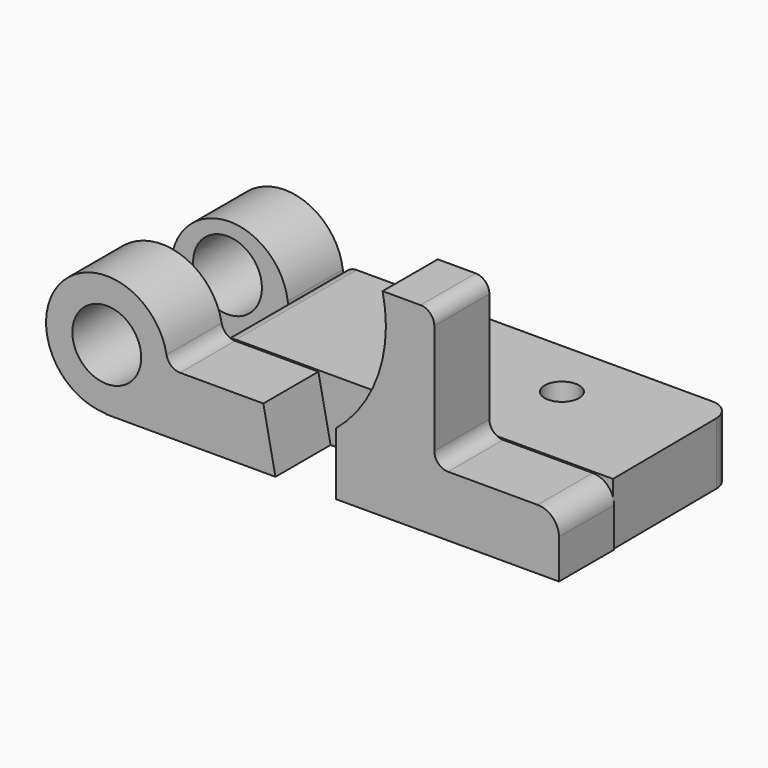
from build123d import *

# Parameters (mm, degrees)
F1_DEPTH      = 25.4
F2_R          = 22.395901736
F3_DEPTH      = 25.4
F5_DEPTH      = 22.86
F6_R          = 6.35
F7_DEPTH      = 22.861
F9_DEPTH      = 25.4
F10_T1_DEPTH  = 25.4
F10_T3_DEPTH  = 50.8
F11_R         = 21.59
F12_DEPTH     = 25.4
F13_T4_DEPTH  = 68.3456632912
F13_S5_R      = 21.59
F13_T6_DEPTH  = 36
F13_T11_DEPTH = 68.3456632912
F13_S12_R     = 21.59
F13_T13_DEPTH = 36
F13_T18_DEPTH = 68.3456632912
F13_S19_R     = 21.59
F13_T20_DEPTH = 36
F14_R         = 12.7
F15_DEPTH     = 81.0466632912


# Not quite as in the source:
# - a fillet or chamfer that OpenCascade refuses, or shapes differently, is made with other operations: its cross-section is extruded or revolved along the edge and cut away or added


with BuildPart() as f1:
    # F0 (on Front) → F1 (new body)
    with BuildSketch(Plane.XZ):
        with BuildLine():
            Line((-62.5702434896, 0), (104.5470208636, 0))
            Line((104.5470208636, 0), (104.5470208636, 14.478))
            ThreePointArc((104.5470208636, 14.478), (102.2407796587, 20.0457587951), (96.6730208636, 22.352))
            Line((96.6730208636, 22.352), (58.5730208636, 22.352))
            Line((58.5730208636, 22.352), (58.5730208636, 73.152))
            Line((58.5730208636, 73.152), (39.5230208636, 73.152))
            ThreePointArc((39.5230208636, 73.152), (37.7930667188, 45.1601637849), (21.4736518763, 22.352))
            Line((21.4736518763, 22.352), (-62.5702434896, 22.352))
            Line((-62.5702434896, 22.352), (-62.5702434896, 0))
        make_face()
    extrude(amount=F1_DEPTH)

    # F2 (on Front) → F3 (join)
    with BuildSketch(Plane.XZ):
        with Locations((-62.223136425, 22.609276697)):
            Circle(F2_R)
    extrude(amount=F3_DEPTH)

    # F4 (on Top) → F5 (join)
    with BuildSketch(Plane.XY):
        with BuildLine():
            Line((-40.0024205446, 55.6456632912), (-40.0024205446, 0))
            Line((-40.0024205446, 0), (104.1451707114, 0))
            Line((104.1451707114, 0), (103.7883380443, 48.0822120633))
            ThreePointArc((103.7883380443, 48.0822120633), (101.536671306, 53.4337730184), (96.1685478742, 55.6456632912))
            Line((96.1685478742, 55.6456632912), (-40.0024205446, 55.6456632912))
        make_face()
    extrude(amount=F5_DEPTH)

    # F6 (on face) → F7 (cut, through all)
    with BuildSketch(Plane.XY.offset(22.86)):
        with Locations((58.6848433214, 33.2936632912)):
            Circle(F6_R)
    extrude(amount=-F7_DEPTH, mode=Mode.SUBTRACT)

    # F8 (on face) → F9 (cut)
    with BuildSketch(Plane.XZ.offset(25.4)):
        with BuildLine():
            Line((22.2823120117, 0), (22.2823120117, 23.0063465614))
            ThreePointArc((22.2823120117, 23.0063465614), (21.8796568843, 22.6771033417), (21.4736518763, 22.352))
            Line((21.4736518763, 22.352), (-4.4883051887, 22.352))
            Line((-4.4883051887, 22.352), (0, 0))
            Line((0, 0), (22.2823120117, 0))
        make_face()
    extrude(amount=-F9_DEPTH, mode=Mode.SUBTRACT)

    # F10: fillet of radius 5.08 on 3 edges, made by hand

    # F10_s2 → F10_t1 (join)
    with BuildSketch(Plane.XZ):
        with BuildLine():
            ThreePointArc((63.6530208636, 22.352), (60.0609184152, 23.8398975516), (58.5730208636, 27.432))
            Line((58.5730208636, 27.432), (58.5730208636, 22.352))
            Line((58.5730208636, 22.352), (63.6530208636, 22.352))
        make_face()
        with BuildLine():
            ThreePointArc((-40.1749339209, 26.5403301063), (-38.4354512238, 23.537383006), (-35.1738015691, 22.352))
            Line((-35.1738015691, 22.352), (-39.8287124925, 22.352))
            ThreePointArc((-39.8287124925, 22.352), (-39.9033629402, 24.4543041094), (-40.1749339209, 26.5403301063))
        make_face()
    extrude(amount=F10_T1_DEPTH)

    # F10_s4 → F10_t3 (cut)
    with BuildSketch(Plane.XZ.offset(-12.7)):
        with BuildLine():
            ThreePointArc((58.5730208636, 68.072), (57.085123312, 71.6641024484), (53.4930208636, 73.152))
            Line((53.4930208636, 73.152), (58.5730208636, 73.152))
            Line((58.5730208636, 73.152), (58.5730208636, 68.072))
        make_face()
    extrude(amount=F10_T3_DEPTH, mode=Mode.SUBTRACT)

    # F11 (on face) → F12 (join)
    with BuildSketch(Plane(origin=(0, 55.6456632912, 0), x_dir=(-1, 0, 0), z_dir=(0, 1, 0))):
        with Locations((61.4217809885, 18.6838455159)):
            Circle(F11_R)
    extrude(amount=-F12_DEPTH)

    # F13: fillet of radius 5.08 on 1 edges, made by hand


with BuildPart() as f13_tool2:
    # F13_s3 → F13_t4 (new body)
    with BuildSketch(Plane.XZ.offset(-68.3456632912)):
        with BuildLine():
            ThreePointArc((-40.0024205446, 17.78), (-38.5145229931, 21.3721024484), (-34.9224205446, 22.86))
            Line((-34.9224205446, 22.86), (-40.0024205446, 22.86))
            Line((-40.0024205446, 22.86), (-40.0024205446, 17.78))
        make_face()
    extrude(amount=F13_T4_DEPTH)

    # F13_s5 → F13_t6 (cut, symmetric)
    with BuildSketch(Plane.XZ.offset(-34.2)):
        with Locations((-61.4217809885, 18.6838455159)):
            Circle(F13_S5_R)
    extrude(amount=F13_T6_DEPTH, both=True, mode=Mode.SUBTRACT)

    split(bisect_by=Plane.XZ.offset(-30.2456632912), keep=Keep.BOTTOM)


with BuildPart() as f1_1:
    add(f1.part)

    # F13_t1: cut F13_tool2
    add(f13_tool2.part, mode=Mode.SUBTRACT)


with BuildPart() as f13_tool9:
    # F13_s10 → F13_t11 (new body)
    with BuildSketch(Plane.XZ.offset(-68.3456632912)):
        with BuildLine():
            ThreePointArc((-40.0024205446, 17.78), (-38.5145229931, 21.3721024484), (-34.9224205446, 22.86))
            Line((-34.9224205446, 22.86), (-40.0024205446, 22.86))
            Line((-40.0024205446, 22.86), (-40.0024205446, 17.78))
        make_face()
    extrude(amount=F13_T11_DEPTH)

    # F13_s12 → F13_t13 (intersect, symmetric)
    with BuildSketch(Plane.XZ.offset(-34.2)):
        with Locations((-61.4217809885, 18.6838455159)):
            Circle(F13_S12_R)
    extrude(amount=F13_T13_DEPTH, both=True, mode=Mode.INTERSECT)

    split(bisect_by=Plane.XZ.offset(-30.2456632912), keep=Keep.TOP)


with BuildPart() as f1_2:
    add(f1_1.part)

    # F13_t8: cut F13_tool9
    add(f13_tool9.part, mode=Mode.SUBTRACT)


with BuildPart() as f13_tool16:
    # F13_s17 → F13_t18 (new body)
    with BuildSketch(Plane.XZ.offset(-68.3456632912)):
        with BuildLine():
            ThreePointArc((-40.0024205446, 17.78), (-38.5145229931, 21.3721024484), (-34.9224205446, 22.86))
            Line((-34.9224205446, 22.86), (-40.0024205446, 22.86))
            Line((-40.0024205446, 22.86), (-40.0024205446, 17.78))
        make_face()
    extrude(amount=F13_T18_DEPTH)

    # F13_s19 → F13_t20 (cut, symmetric)
    with BuildSketch(Plane.XZ.offset(-34.2)):
        with Locations((-61.4217809885, 18.6838455159)):
            Circle(F13_S19_R)
    extrude(amount=F13_T20_DEPTH, both=True, mode=Mode.SUBTRACT)

    split(bisect_by=Plane.XZ.offset(-30.2456632912), keep=Keep.TOP)


with BuildPart() as f1_3:
    add(f1_2.part)

    # F13_t15: cut F13_tool16
    add(f13_tool16.part, mode=Mode.SUBTRACT)

    # F14 (on face) → F15 (cut, through all)
    with BuildSketch(Plane.XZ.offset(25.4)):
        with Locations((-62.223136425, 22.609276697)):
            Circle(F14_R)
    extrude(amount=-F15_DEPTH, mode=Mode.SUBTRACT)


solid = f1_3.part
